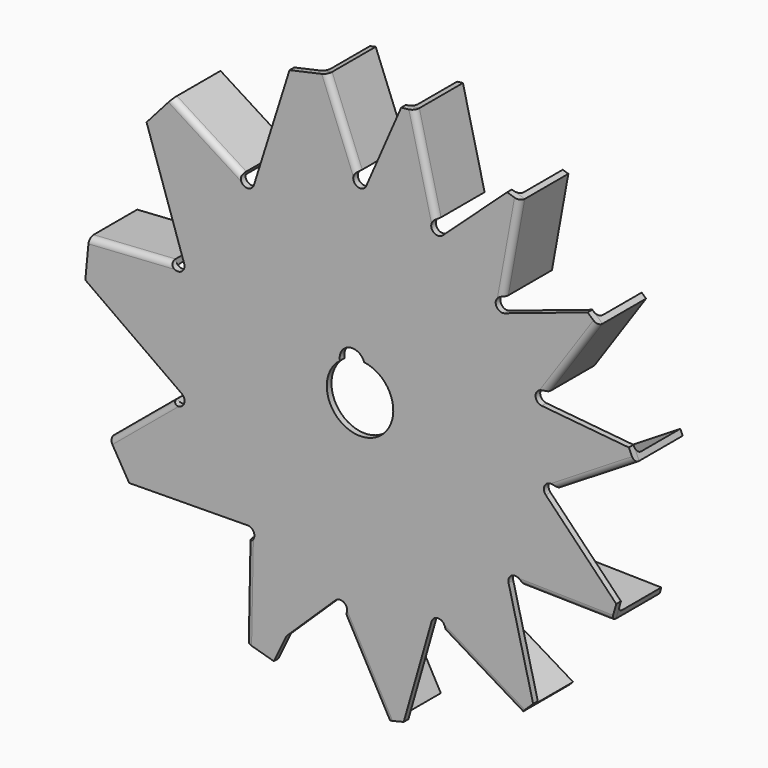
from build123d import *

# Parameters (mm, degrees)
F1_DEPTH = 1.5
F3_DEPTH = 15.5
F4_R     = 1.5
F5_R     = 1.5


# Not quite as in the source:
# - ends of sketch curves that miss each other by under 0.0002 mm in the source are joined


with BuildPart() as f1:
    # F0 (on Front) → F1 (new body)
    with BuildSketch(Plane.XZ):
        with BuildLine():
            ThreePointArc((1.604855, 48.602189), (-1.258921, 48.084427), (-0.641172, 50.928311))
            Line((-0.641172, 50.928311), (-8.369604, 70.555313))
            Line((-8.369604, 70.555313), (-18.133274, 68.394123))
            Line((-18.133274, 68.394123), (-27.295885, 39.367266))
            ThreePointArc((-27.295885, 39.367266), (-29.702564, 38.307202), (-30.443013, 40.830607))
            Line((-30.443013, 40.830607), (-48.276929, 52.129077))
            Line((-48.276929, 52.129077), (-54.900645, 44.637322))
            Line((-54.900645, 44.637322), (-45.232748, 15.774838))
            ThreePointArc((-45.232748, 15.774838), (-46.555202, 13.501746), (-48.638518, 15.106622))
            Line((-48.638518, 15.106622), (-69.706646, 13.750854))
            Line((-69.706646, 13.750854), (-70.655233, 3.795946))
            Line((-70.655233, 3.795946), (-45.857151, -13.855279))
            ThreePointArc((-45.857151, -13.855279), (-45.589221, -16.471393), (-48.21803, -16.399298))
            Line((-48.21803, -16.399298), (-64.456703, -29.890398))
            Line((-64.456703, -29.890398), (-59.367096, -38.498296))
            Line((-59.367096, -38.498296), (-28.930108, -38.182404))
            ThreePointArc((-28.930108, -38.182404), (-27.161963, -39.93982), (-28.945126, -41.681995))
            Line((-28.945126, -41.681995), (-29.381429, -64.690294))
            Line((-29.381429, -64.690294), (-22.169409, -66.748635))
            Line((-22.169409, -66.748635), (-18.960605, -60.026149))
            Line((-18.960605, -60.026149), (-6.309677, -47.778944))
            ThreePointArc((-6.309677, -47.778944), (-3.685363, -47.995817), (-4.246986, -50.568489))
            Line((-4.246986, -50.568489), (6.871037, -70.716981))
            Line((6.871037, -70.716981), (11.236464, -69.624713))
            Line((11.236464, -69.624713), (18.406841, -44.540181))
            ThreePointArc((18.406841, -44.540181), (20.788462, -43.41682), (21.587388, -45.925959))
            Line((21.587388, -45.925959), (41.285235, -57.824146))
            Line((41.285235, -57.824146), (44.520957, -54.696831))
            Line((44.520957, -54.696831), (38.198817, -29.385197))
            ThreePointArc((38.198817, -29.385197), (39.700571, -27.222144), (41.646301, -28.99646))
            Line((41.646301, -28.99646), (64.654039, -29.461122))
            Line((64.654039, -29.461122), (65.894376, -25.135435))
            Line((65.894376, -25.135435), (47.771133, -6.368538))
            ThreePointArc((47.771133, -6.368538), (47.956335, -3.770918), (50.519107, -4.233655))
            Line((50.519107, -4.233655), (70.580991, 8.150225))
            Line((70.580991, 8.150225), (69.129548, 11.335082))
            Line((69.129548, 11.335082), (46.719275, 13.492864))
            ThreePointArc((46.719275, 13.492864), (45.241564, 15.830666), (47.873515, 16.680244))
            Line((47.873515, 16.680244), (61.16401, 36.153373))
            Line((61.16401, 36.153373), (58.542657, 38.472534))
            Line((58.542657, 38.472534), (37.1922, 31.328715))
            ThreePointArc((37.1922, 31.328715), (34.891377, 32.863367), (36.950231, 34.710003))
            Line((36.950231, 34.710003), (41.171299, 57.905325))
            Line((41.171299, 57.905325), (37.833288, 58.957789))
            Line((37.833288, 58.957789), (21.234314, 43.747596))
            ThreePointArc((21.234314, 43.747596), (18.508209, 44.213745), (19.637974, 46.738141))
            Line((19.637974, 46.738141), (14.059753, 69.644999))
            Line((14.059753, 69.644999), (10.582252, 69.248787))
            Line((10.582252, 69.248787), (1.604855, 48.602189))
        make_face()
        with BuildLine():
            ThreePointArc((1.085106, 8.480863), (2.212903, -8.258666), (-5.180161, 6.80209))
            ThreePointArc((-5.180161, 6.80209), (-2.834069, 10.576888), (1.085106, 8.480863))
        make_face(mode=Mode.SUBTRACT)
    extrude(amount=F1_DEPTH)

    # F2 (on face) → F3 (join)
    with BuildSketch(Plane.XZ.offset(1.5)):
        Polygon((-30.443013, 40.830607), (-48.276929, 52.129077), (-49.283222, 50.990909), (-31.245777, 39.563496), align=None)
        Polygon((-0.641172, 50.928311), (-8.369604, 70.555313), (-9.852458, 70.227083), (-2.036867, 50.378735), align=None)
        Polygon((19.637974, 46.738141), (14.059753, 69.644999), (12.557596, 69.473849), (18.180564, 46.383236), align=None)
        Polygon((36.950231, 34.710003), (41.171299, 57.905325), (39.729397, 58.359952), (35.474468, 34.978561), align=None)
        Polygon((47.873515, 16.680244), (61.16401, 36.153373), (60.031679, 37.155168), (46.63457, 17.525829), align=None)
        Polygon((50.519107, -4.233655), (70.580991, 8.150225), (69.954019, 9.52597), (49.731203, -2.957251), align=None)
        Polygon((41.646301, -28.99646), (64.654039, -29.461122), (65.081756, -27.969454), (41.676589, -27.496766), align=None)
        Polygon((21.587388, -45.925959), (41.285235, -57.824146), (42.40104, -56.745724), (22.362937, -44.642011), align=None)
        Polygon((-4.246986, -50.568489), (6.871037, -70.716981), (8.376409, -70.340324), (-2.933664, -49.843793), align=None)
        Polygon((-28.945126, -41.681995), (-29.381429, -64.690294), (-27.889235, -65.116172), (-27.445396, -41.710435), align=None)
        Polygon((-48.21803, -16.399298), (-64.456703, -29.890398), (-63.683476, -31.198133), (-47.259479, -17.553066), align=None)
        Polygon((-48.638518, 15.106622), (-69.706646, 13.750854), (-69.850758, 12.238478), (-48.54219, 13.609718), align=None)
    extrude(amount=-F3_DEPTH)

    # F4
    f4_edges = [f1.edges().sort_by_distance(p)[0] for p in [
        (-5.944663, 0, 60.302909),
        (-40.264499, 0, 45.277203),
        (-59.196474, 0, 12.924098),
        (-55.471478, 0, -24.3756),
        (-27.667315, 0, -53.413304),
        (2.721372, 0, -60.092058),
        (32.381989, 0, -50.693867),
        (53.379173, 0, -27.73311),
        (59.842611, 0, 3.28436),
        (53.333124, 0, 27.340499),
        (37.601932, 0, 46.669257),
        (15.36908, 0, 57.928543),
    ]]
    fillet(f4_edges, radius=F4_R)

    # F5
    f5_edges = [f1.edges().sort_by_distance(p)[0] for p in [
        (-4.505388, -1.5, 60.741812),
        (16.848863, -1.5, 58.19157),
        (39.060765, -1.5, 46.307664),
        (54.518762, -1.5, 26.416808),
        (60.550049, -1.5, 1.958285),
        (53.15017, -1.5, -29.228791),
        (31.436311, -1.5, -51.875052),
        (1.312026, -1.5, -60.642735),
        (-29.163278, -1.5, -53.186145),
        (-56.337367, -1.5, -23.144848),
        (-59.172582, -1.5, 14.428738),
        (-39.359971, -1.5, 46.479842),
    ]]
    fillet(f5_edges, radius=F5_R)


solid = f1.part
